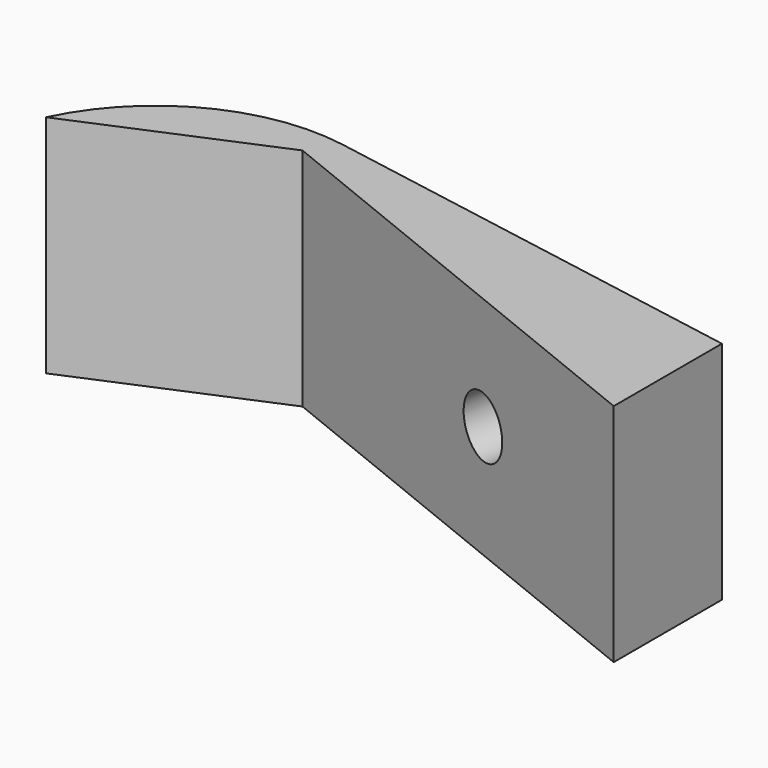
from build123d import *

# Parameters (mm, degrees)
F1_DEPTH    = 15
F2_T1_DEPTH = 86.0591430992
F3_R        = 2
F4_DEPTH    = 16.3887129303
F5_R        = 3.5
F5_R_2      = 2
F6_DEPTH    = 3


# Not quite as in the source:
# - a fillet or chamfer that OpenCascade refuses, or shapes differently, is made with other operations: its cross-section is extruded or revolved along the edge and cut away or added


with BuildPart() as f1:
    # F0 (on Top) → F1 (new body)
    with BuildSketch(Plane.XY):
        Polygon((-12.7344739318, -5.4054634817), (0, 0), (30.5970672007, -12.3620175827), (30.5970672007, -3.3620175827), (-12.7344739318, 4.2785022346), align=None)
    extrude(amount=F1_DEPTH)

    # F2: fillet of radius 13 on 1 edges, made by hand

    # F2_s2 → F2_t1 (cut)
    with BuildSketch(Plane.XY.offset(-35.5295715496)):
        with BuildLine():
            ThreePointArc((-12.7344739318, -5.4054634817), (-6.9533889828, 0.5627654484), (1.2614450775, 1.8106440935))
            Line((1.2614450775, 1.8106440935), (-12.7344739318, 4.2785022346))
            Line((-12.7344739318, 4.2785022346), (-12.7344739318, -5.4054634817))
        make_face()
    extrude(amount=F2_T1_DEPTH, mode=Mode.SUBTRACT)

    # F3 (on face) → F4 (cut, through all)
    with BuildSketch(Plane(origin=(0.3476755995, 1.9717663066, 0), x_dir=(-0.984807753, 0.1736481777, 0), z_dir=(0.1736481777, 0.984807753, 0))):
        with Locations((-18.7160372252, 7.5)):
            Circle(F3_R)
    extrude(amount=-F4_DEPTH, mode=Mode.SUBTRACT)

    # F5 (on face) → F6 (cut)
    with BuildSketch(Plane(origin=(0.3476755995, 1.9717663066, 0), x_dir=(-0.984807753, 0.1736481777, 0), z_dir=(0.1736481777, 0.984807753, 0))):
        with Locations((-18.7160372252, 7.5)):
            Circle(F5_R)
        with Locations((-18.7160372252, 7.5)):
            Circle(F5_R_2, mode=Mode.SUBTRACT)
    extrude(amount=-F6_DEPTH, mode=Mode.SUBTRACT)


solid = f1.part
